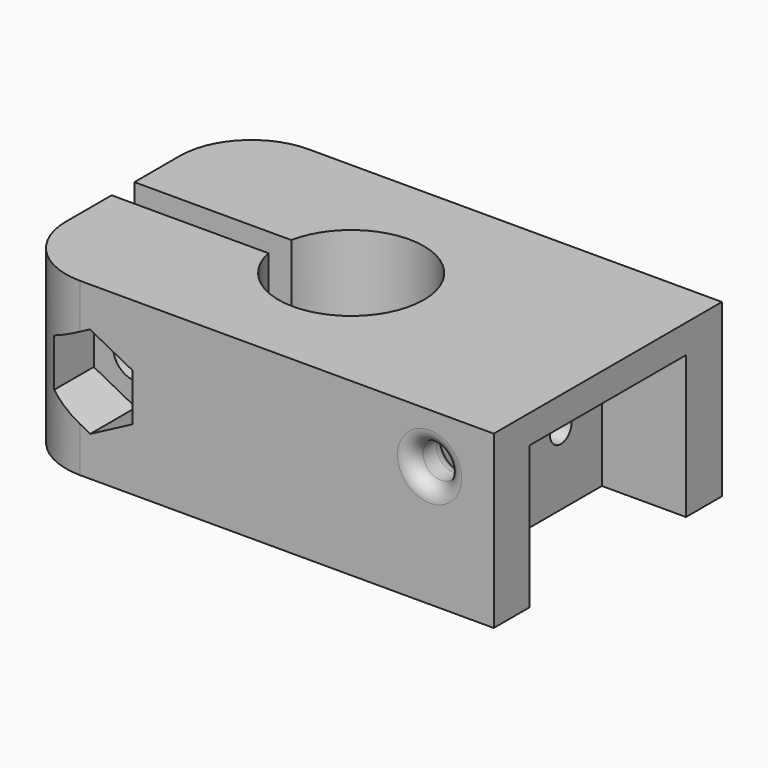
from build123d import *

# Parameters (mm, degrees)
F1_DEPTH     = 12
F2_W         = 5.9
F2_H         = 13.7
F3_DEPTH     = 10
F4_R         = 1.6
F5_DEPTH     = 20.001
F6_R         = 1.25
F7_DEPTH     = 16
F9_R         = 0.95
F10_DEPTH    = 7
F11_R        = 1.6
F12_DEPTH    = 4
F13_R        = 2.8
F14_DEPTH    = 3
F15_T1_DEPTH = 37


# Not quite as in the source:
# - a fillet or chamfer that OpenCascade refuses, or shapes differently, is made with other operations: its cross-section is extruded or revolved along the edge and cut away or added


with BuildPart() as f1:
    # F0 (on Top) → F1 (new body)
    with BuildSketch(Plane.XY):
        with BuildLine():
            Line((18, 10), (-16, 10))
            Line((-16, 10), (-16, 1))
            Line((-16, 1), (-5.0009999, 1))
            ThreePointArc((-5.0009999, 1), (5.1, 0), (-5.0009999, -1))
            Line((-5.0009999, -1), (-16, -1))
            Line((-16, -1), (-16, -10))
            Line((-16, -10), (18, -10))
            Line((18, -10), (18, -6.85))
            Line((18, -6.85), (18, 6.85))
            Line((18, 6.85), (18, 10))
        make_face()
    extrude(amount=F1_DEPTH)

    # F2 (on face) → F3 (cut)
    with BuildSketch(Plane(origin=(0, 0, 0), x_dir=(1, 0, 0), z_dir=(0, 0, -1))):
        with Locations((15.05, 0)):
            Rectangle(F2_W, F2_H)
    extrude(amount=-F3_DEPTH, mode=Mode.SUBTRACT)

    # F4 (on face) → F5 (cut, through all)
    with BuildSketch(Plane.XZ.offset(10)):
        with Locations((-10.3, 6)):
            Circle(F4_R)
    extrude(amount=-F5_DEPTH, mode=Mode.SUBTRACT)

    # F6 (on face) → F7 (cut)
    with BuildSketch(Plane.XZ.offset(10)):
        with Locations((13.5, 8.5)):
            Circle(F6_R)
    extrude(amount=-F7_DEPTH, mode=Mode.SUBTRACT)

    # F8: fillet of radius 1 on 2 edges, made by hand

    # F8_s1 → F8_t2 (revolve, cut)
    with BuildSketch(Plane.XY.offset(8.5)):
        with BuildLine():
            ThreePointArc((15.75, -10), (15.0428932188, -9.7071067812), (14.75, -9))
            Line((14.75, -9), (14.75, -10))
            Line((14.75, -10), (15.75, -10))
        make_face()
    revolve(axis=Axis((13.5, -10, 8.5), (0, -1, 0)), mode=Mode.SUBTRACT)


with BuildPart() as f8_tool4:
    # F8_s5 → F8_t6 (revolve)
    with BuildSketch(Plane.XY.offset(8.5)):
        with BuildLine():
            ThreePointArc((15.75, -6.85), (15.0428932188, -7.1428932188), (14.75, -7.85))
            Line((14.75, -7.85), (14.75, -6.85))
            Line((14.75, -6.85), (15.75, -6.85))
        make_face()
    revolve(axis=Axis((13.5, -6.85, 8.5), (0, -1, 0)))

    split(bisect_by=Plane.XY.offset(10), keep=Keep.BOTTOM)

    split(bisect_by=Plane.YZ.offset(12.1), keep=Keep.TOP)


with BuildPart() as f1_1:
    add(f1.part)

    # F8_t3: cut F8_tool4
    add(f8_tool4.part, mode=Mode.SUBTRACT)

    # F9 (on face) → F10 (cut)
    with BuildSketch(Plane.YZ.offset(12.1)):
        with Locations((46.374425292, 0.8309943862)):
            Circle(F9_R)
        with Locations((46.374425292, -5.6690056138)):
            Circle(F9_R)
        with Locations((-3.25, 5)):
            Circle(F9_R)
        with Locations((3.25, 5)):
            Circle(F9_R)
    extrude(amount=-F10_DEPTH, mode=Mode.SUBTRACT)

    # F11 (on face) → F12 (cut)
    with BuildSketch(Plane.XZ.offset(10)):
        Polygon((-7.35, 7.6736242323), (-10.3143082515, 9.227305642), (-13.25, 7.6886229858), (-13.25, 4.3268273558), (-10.3, 2.7806453228), (-7.35, 4.3268273558), align=None)
        with Locations((-10.3, 6)):
            Circle(F11_R, mode=Mode.SUBTRACT)
    extrude(amount=-F12_DEPTH, mode=Mode.SUBTRACT)

    # F13 (on face) → F14 (cut)
    with BuildSketch(Plane(origin=(0, 10, 0), x_dir=(-1, 0, 0), z_dir=(0, 1, 0))):
        with Locations((10.3, 6)):
            Circle(F13_R)
    extrude(amount=-F14_DEPTH, mode=Mode.SUBTRACT)

    # F15: fillet of radius 5 on 2 edges, made by hand

    # F15_s2 → F15_t1 (cut)
    with BuildSketch(Plane.XY.offset(-12.5)):
        with BuildLine():
            ThreePointArc((-11, -10), (-14.5355339059, -8.5355339059), (-16, -5))
            Line((-16, -5), (-16, -10))
            Line((-16, -10), (-11, -10))
        make_face()
        with BuildLine():
            ThreePointArc((-11, 10), (-14.5355339059, 8.5355339059), (-16, 5))
            Line((-16, 5), (-16, 10))
            Line((-16, 10), (-11, 10))
        make_face()
    extrude(amount=F15_T1_DEPTH, mode=Mode.SUBTRACT)


solid = f1_1.part
